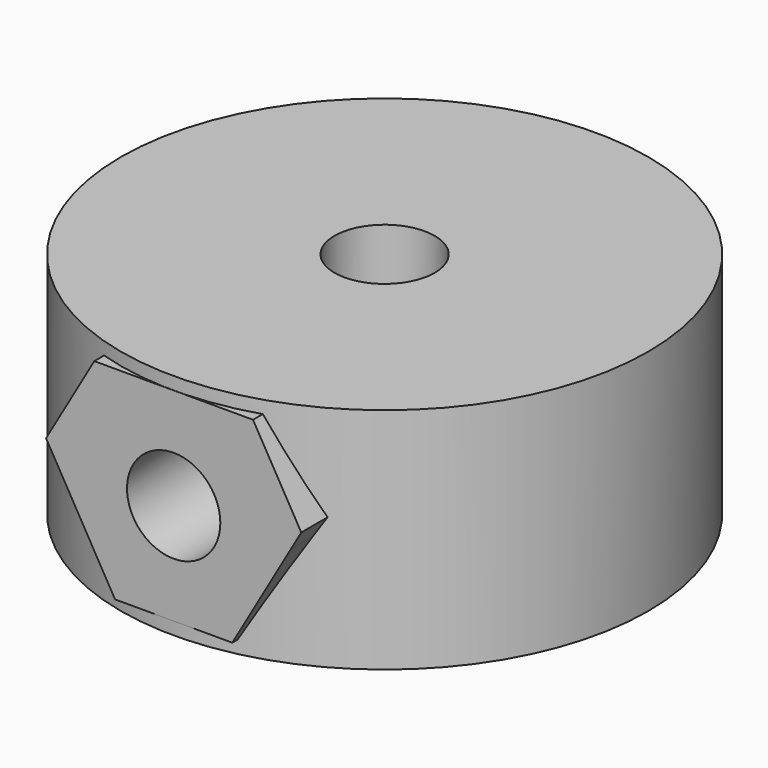
from build123d import *

# Parameters (mm, degrees)
F0_R           = 12.7
F0_R_2         = 3.4925
F1_DEPTH       = 5.5
F3_R           = 2.2479
F4_DEPTH       = 7.62
F6_DEPTH       = 7.62
F7_DEPTH       = 4.42
F8_DEPTH       = 12.7
F9_R           = 4.1894842837
F9_R_2         = 2.413
F10_DEPTH      = 5.5
F10_DEPTH_BACK = 2.5


with BuildPart() as f1:
    # F0 (on Top) → F1 (new body, symmetric)
    with BuildSketch(Plane.XY):
        Circle(F0_R)
        Circle(F0_R_2, mode=Mode.SUBTRACT)
    extrude(amount=F1_DEPTH, both=True)

    # F3 (on offset) → F4 (cut)
    with BuildSketch(Plane.XZ.offset(12.7)):
        Circle(F3_R)
    extrude(amount=-F4_DEPTH, mode=Mode.SUBTRACT)

    # F5 (on offset) → F6 (cut)
    with BuildSketch(Plane.XZ.offset(12.7)):
        Polygon((-6.1459082824, 0.8660254038), (-5.6459082824, 0), (-2.8229541412, 4.8895), (-3.8229541412, 4.8895), align=None)
        Polygon((-2.8229541412, -4.8895), (2.8229541412, -4.8895), (5.6459082824, 0), (2.8229541412, 4.8895), (-2.8229541412, 4.8895), (-5.6459082824, 0), align=None)
        Polygon((2.8229541412, 4.8895), (5.6459082824, 0), (6.1459082824, 0.8660254038), (3.8229541412, 4.8895), align=None)
    extrude(amount=-F6_DEPTH, mode=Mode.SUBTRACT)

    # F9 (on Top) → F10 (join, two sides)
    with BuildSketch(Plane.XY) as f10_sk:
        Circle(F9_R)
        Circle(F9_R_2, mode=Mode.SUBTRACT)
    extrude(amount=F10_DEPTH)
    extrude(f10_sk.sketch, amount=-F10_DEPTH_BACK)


with BuildPart() as f7:
    # F5 (on offset) → F7 (new body)
    with BuildSketch(Plane.XZ.offset(12.7)):
        Polygon((-2.8229541412, -4.8895), (2.8229541412, -4.8895), (5.6459082824, 0), (2.8229541412, 4.8895), (-2.8229541412, 4.8895), (-5.6459082824, 0), align=None)
        Polygon((2.8229541412, 4.8895), (5.6459082824, 0), (6.1459082824, 0.8660254038), (3.8229541412, 4.8895), align=None)
        Polygon((-6.1459082824, 0.8660254038), (-5.6459082824, 0), (-2.8229541412, 4.8895), (-3.8229541412, 4.8895), align=None)
    extrude(amount=-F7_DEPTH)

    # F3 (on offset) → F8 (cut)
    with BuildSketch(Plane.XZ.offset(12.7)):
        Circle(F3_R)
    extrude(amount=-F8_DEPTH, mode=Mode.SUBTRACT)


solid = Compound([f1.part, f7.part])
